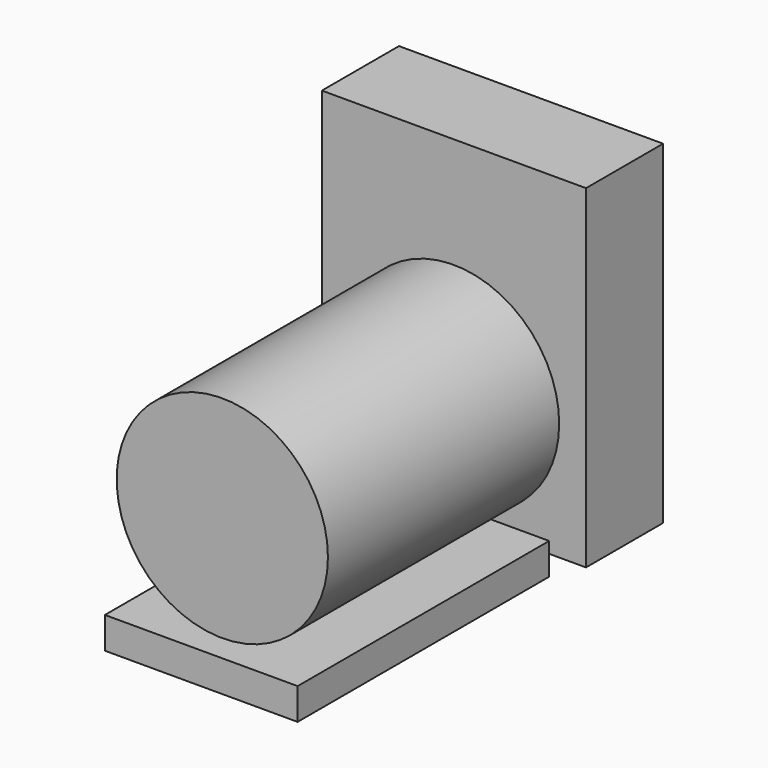
from build123d import *

# Parameters (mm, degrees)
F0_R     = 27.8422041497
F1_DEPTH = 101.6
F2_W     = 69.6255154908
F2_H     = 88.0208928138
F3_DEPTH = 25.4
F4_W     = 82.8780960292
F4_H     = 8.307589218
F5_DEPTH = 25.4
F6_DEPTH = 25.4


# Not quite as in the source:
# - the program builds the solid bodies; features that only make, move or delete a surface that nothing else refers to are left out


with BuildPart() as f1:
    # F0 (on Front) → F1 (new body)
    with BuildSketch(Plane.XZ):
        Circle(F0_R)
    extrude(amount=F1_DEPTH)

    # F2 (on Front) → F3 (join)
    with BuildSketch(Plane.XZ):
        with Locations((0.0989008695, 12.9558844492)):
            Rectangle(F2_W, F2_H)
    extrude(amount=F3_DEPTH)


with BuildPart() as f5:
    # F4 (on Right) → F5 (new body)
    with BuildSketch(Plane.YZ):
        with Locations((-67.0949304476, -32.0435585454)):
            Rectangle(F4_W, F4_H)
    extrude(amount=F5_DEPTH)

    # F6 (add): a face of the model
    f6_faces = [f5.faces().sort_by_distance(p)[0] for p in [
        (0, -67.0949304476, -32.0435585454),
    ]]
    extrude(f6_faces, amount=F6_DEPTH)


solid = Compound([f1.part, f5.part])
